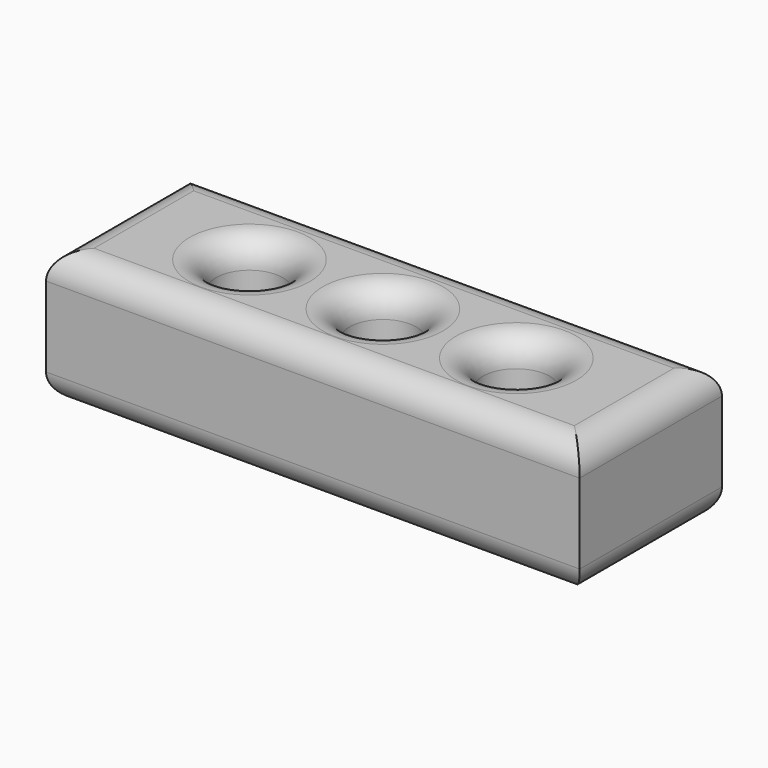
from build123d import *

# Parameters (mm, degrees)
F0_W     = 50.8
F0_H     = 16.92773588
F1_DEPTH = 12.7
F2_R     = 3.175
F3_DEPTH = 25.4
F4_R     = 2.54
F5_R     = 2.54


with BuildPart() as f1:
    # F0 (on Top) → F1 (new body)
    with BuildSketch(Plane.XY):
        with Locations((0, 0.1322478056)):
            Rectangle(F0_W, F0_H)
    extrude(amount=F1_DEPTH)

    # F2 (on face) → F3 (cut)
    with BuildSketch(Plane.XY.offset(12.7)):
        with Locations((-12.7, 0)):
            Circle(F2_R)
        Circle(F2_R)
        with Locations((12.7, 0)):
            Circle(F2_R)
    extrude(amount=-F3_DEPTH, mode=Mode.SUBTRACT)

    # F4
    f4_edges = [f1.edges().sort_by_distance(p)[0] for p in [
        (-15.875, 0, 12.7),
        (-3.175, 0, 12.7),
        (9.525, 0, 12.7),
        (-15.875, 0, 0),
        (-3.175, 0, 0),
        (9.525, 0, 0),
    ]]
    fillet(f4_edges, radius=F4_R)

    # F5
    f5_edges = [f1.edges().sort_by_distance(p)[0] for p in [
        (0, 8.596116, 12.7),
        (25.4, 0.132248, 12.7),
        (0, -8.33162, 12.7),
        (-25.4, 0.132248, 12.7),
        (0, 8.596116, 0),
        (-25.4, 0.132248, 0),
        (0, -8.33162, 0),
        (25.4, 0.132248, 0),
    ]]
    fillet(f5_edges, radius=F5_R)


solid = f1.part
